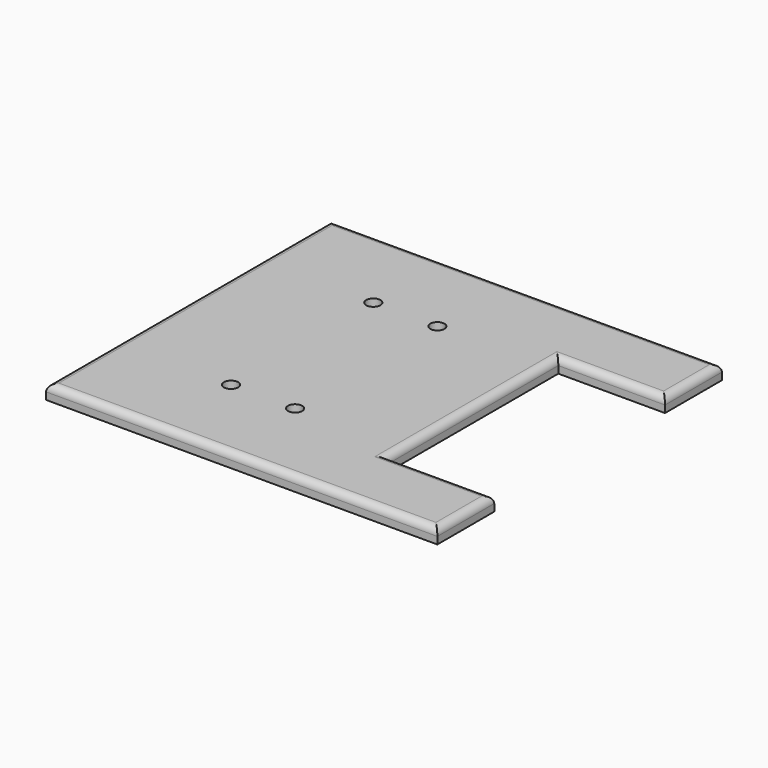
from build123d import *

# Parameters (mm, degrees)
F0_R     = 1
F0_W     = 15
F0_H     = 10
F1_DEPTH = 2
F2_R     = 1


# Not quite as in the source:
# - a feature names something its author has since deleted; it is built from what else it names


with BuildPart() as f1:
    # F0 (on Top) → F1 (new body)
    with BuildSketch(Plane.XY):
        Polygon((-20, -25), (20, -25), (20, -15), (20, 15), (20, 25), (-20, 25), align=None)
        with Locations((-4, -12.5)):
            Circle(F0_R, mode=Mode.SUBTRACT)
        with Locations((5, -12.5)):
            Circle(F0_R, mode=Mode.SUBTRACT)
        with Locations((-4, 12.5)):
            Circle(F0_R, mode=Mode.SUBTRACT)
        with Locations((5, 12.5)):
            Circle(F0_R, mode=Mode.SUBTRACT)
        with Locations((27.5, -20)):
            Rectangle(F0_W, F0_H)
        with Locations((27.5, 20)):
            Rectangle(F0_W, F0_H)
    extrude(amount=-F1_DEPTH)

    # F2
    f2_edges = [f1.edges().sort_by_distance(p)[0] for p in [
        (7.5, 25, 0),
        (-20, 0, 0),
        (35, 20, 0),
        (27.5, 15, 0),
        (20, 0, 0),
        (27.5, -15, 0),
        (35, -20, 0),
        (7.5, -25, 0),
    ]]
    fillet(f2_edges, radius=F2_R)


solid = f1.part
